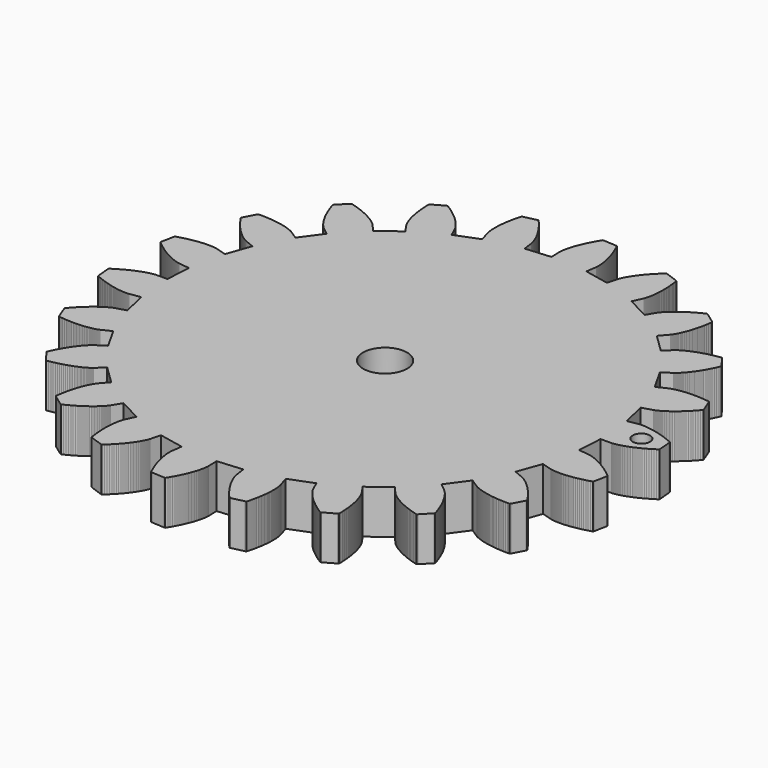
from build123d import *

# Parameters (mm, degrees)
F0_R     = 2.5
F1_DEPTH = 5


# Not quite as in the source:
# - the dataset's text gives a spline's control points without its knots; the knots are read off the source's solid


with BuildPart() as f1:
    # F0 (on Top) → F1 (new body)
    with BuildSketch(Plane.XY):
        Polygon((26.3997478077, -0.4197545319), (26.5654568077, 2.4303734681), (27.7857098077, 2.4303734681), (27.7960448077, 2.4307174681), (27.8132698077, 2.4314064681), (27.8363528077, 2.4327844681), (27.8663248077, 2.4348524681), (27.9024978077, 2.4382974681), (27.9452178077, 2.4427754681), (27.9944818077, 2.4486324681), (28.0499478077, 2.4562114681), (28.1116158077, 2.4658574681), (28.1794838077, 2.4772264681), (28.2535538077, 2.4910074681), (28.3341688077, 2.5071994681), (28.4202958077, 2.5264914681), (28.5129688077, 2.5481954681), (28.6111548077, 2.5730004681), (28.7155408077, 2.6012504681), (28.8254388077, 2.6326004681), (28.9411948077, 2.6677404681), (29.0628068077, 2.7070144681), (29.1895858077, 2.7500784681), (29.3218778077, 2.7972764681), (29.4596818077, 2.8489524681), (29.6026528077, 2.9051074681), (29.7507918077, 2.9657414681), (29.9037538077, 3.0315424681), (30.0615398077, 3.1025114681), (30.2241478077, 3.1786484681), (30.3912348077, 3.2602964681), (30.5631458077, 3.3474574681), (30.7388448077, 3.4404754681), (30.9193678077, 3.5393494681), (31.1036808077, 3.6440804681), (31.2917828077, 3.7550124681), (31.4840198077, 3.8724904681), (31.6793568077, 3.9965134681), (31.8784828077, 4.1270824681), (31.8850288077, 4.2528284681), (31.7627278077, 5.6880554681), (31.7355118077, 5.8107014681), (31.5170928077, 5.9061304681), (31.3034968077, 5.9950134681), (31.0943788077, 6.0783854681), (30.8900848077, 6.1562444681), (30.6906138077, 6.2285914681), (30.4963108077, 6.2954264681), (30.3071748077, 6.3574374681), (30.1232068077, 6.4142814681), (29.9444058077, 6.4663024681), (29.7714628077, 6.5141894681), (29.6040308077, 6.5572534681), (29.4421118077, 6.5965274681), (29.2857038077, 6.6313224681), (29.1354978077, 6.6626734681), (28.9911488077, 6.6902334681), (28.8526558077, 6.7143494681), (28.7203638077, 6.7353644681), (28.5939288077, 6.7536234681), (28.4740398077, 6.7687824681), (28.3603518077, 6.7811844681), (28.2528648077, 6.7911754681), (28.1515788077, 6.7990994681), (28.0568388077, 6.8049554681), (27.9682998077, 6.8090894681), (27.8863058077, 6.8115014681), (27.8108588077, 6.8128794681), (27.7419568077, 6.8128794681), (27.6796008077, 6.8115014681), (27.6237898077, 6.8097784681), (27.5741808077, 6.8073674681), (27.5314618077, 6.8046114681), (27.4949438077, 6.8018554681), (27.4653158077, 6.7987544681), (27.4418888077, 6.7963424681), (27.4253528077, 6.7939314681), (27.4150168077, 6.7925534681), (26.2119898077, 6.5865364681), (25.5677568077, 9.3681064681), (26.7387448077, 9.7119274681), (26.7487358077, 9.7150274681), (26.7645828077, 9.7205394681), (26.7866318077, 9.7284634681), (26.8148818077, 9.7387984681), (26.8486438077, 9.7522344681), (26.8886068077, 9.7687714681), (26.9337378077, 9.7880634681), (26.9850688077, 9.8111454681), (27.0415688077, 9.8376734681), (27.1035808077, 9.8679904681), (27.1707598077, 9.9020964681), (27.2431068077, 9.9403374681), (27.3206218077, 9.9827114681), (27.4033038077, 10.0299094681), (27.4908088077, 10.0812414681), (27.5827938077, 10.1377414681), (27.6796008077, 10.1990634681), (27.7808858077, 10.2655544681), (27.8863058077, 10.3368674681), (27.9958598077, 10.4140374681), (28.1095488077, 10.4967194681), (28.2270258077, 10.5849144681), (28.3482938077, 10.6789654681), (28.4733508077, 10.7792174681), (28.6015078077, 10.8853264681), (28.7331108077, 10.9979814681), (28.8674698077, 11.1168374681), (29.0049288077, 11.2422384681), (29.1451438077, 11.3741854681), (29.2877708077, 11.5130234681), (29.4331538077, 11.6587504681), (29.5802598077, 11.8110234681), (29.7297768077, 11.9708764681), (29.8810168077, 12.1376184681), (30.0336338077, 12.3115964681), (30.1876298077, 12.4931524681), (30.1583468077, 12.6151094681), (29.6371038077, 13.9583514681), (29.5761258077, 14.0682504681), (29.3397918077, 14.0978784681), (29.1096598077, 14.1233724681), (28.8857288077, 14.1443874681), (28.6676538077, 14.1616124681), (28.4561248077, 14.1747034681), (28.2507978077, 14.1840054681), (28.0516708077, 14.1902064681), (27.8590898077, 14.1929624681), (27.6730548077, 14.1926184681), (27.4935658077, 14.1895174681), (27.3206218077, 14.1840054681), (27.1542238077, 14.1757374681), (26.9947158077, 14.1654024681), (26.8414088077, 14.1529994681), (26.6953368077, 14.1388744681), (26.5554658077, 14.1230274681), (26.4228298077, 14.1058024681), (26.2963948077, 14.0875434681), (26.1768498077, 14.0682504681), (26.0641948077, 14.0482684681), (25.9584308077, 14.0275984681), (25.8588678077, 14.0069274681), (25.7661948077, 13.9855684681), (25.6804118077, 13.9648974681), (25.6011748077, 13.9442274681), (25.5284828077, 13.9239004681), (25.4623368077, 13.9042634681), (25.4027368077, 13.8856604681), (25.3493378077, 13.8680904681), (25.3028288077, 13.8518984681), (25.2625218077, 13.8374294681), (25.2284148077, 13.8243374681), (25.2005098077, 13.8129684681), (25.1791498077, 13.8040114681), (25.1636468077, 13.7971214681), (25.1540008077, 13.7929874681), (24.0577718077, 13.2562414681), (22.6559618077, 15.7436004681), (23.6829448077, 16.4033364681), (23.6915578077, 16.4095374681), (23.7053388077, 16.4191834681), (23.7242868077, 16.4329644681), (23.7480578077, 16.4508784681), (23.7769968077, 16.4732714681), (23.8104138077, 16.5001434681), (23.8486548077, 16.5314934681), (23.8910288077, 16.5680114681), (23.9378818077, 16.6093524681), (23.9888698077, 16.6558614681), (24.0436468077, 16.7075384681), (24.1025578077, 16.7647264681), (24.1649138077, 16.8274274681), (24.2310598077, 16.8956404681), (24.3003068077, 16.9697094681), (24.3726538077, 17.0496364681), (24.4481008077, 17.1357634681), (24.5266488077, 17.2280924681), (24.6076088077, 17.3266214681), (24.6913248077, 17.4313524681), (24.7767628077, 17.5426294681), (24.8649578077, 17.6604514681), (24.9545298077, 17.7848194681), (25.0461698077, 17.9164224681), (25.1395318077, 18.0542254681), (25.2339268077, 18.1992644681), (25.3293568077, 18.3511934681), (25.4261638077, 18.5103564681), (25.5233148077, 18.6764104681), (25.6211558077, 18.8496984681), (25.7193408077, 19.0305664681), (25.8178708077, 19.2183234681), (25.9160558077, 19.4136604681), (26.0142418077, 19.6162324681), (26.1117378077, 19.8263834681), (26.2085448077, 20.0437684681), (26.1461888077, 20.1526334681), (25.2673448077, 21.2943384681), (25.1781168077, 21.3828774681), (24.9428168077, 21.3446364681), (24.7147518077, 21.3043294681), (24.4939208077, 21.2612654681), (24.2799798077, 21.2161344681), (24.0732748077, 21.1692814681), (23.8734588077, 21.1203604681), (23.6808778077, 21.0704074681), (23.4951878077, 21.0187304681), (23.3167318077, 20.9660204681), (23.1455108077, 20.9126214681), (22.9811788077, 20.8581894681), (22.8240828077, 20.8034124681), (22.6735318077, 20.7486354681), (22.5302158077, 20.6938584681), (22.3937908077, 20.6387364681), (22.2642548077, 20.5843044681), (22.1416098077, 20.5305604681), (22.0255098077, 20.4775064681), (21.9166448077, 20.4251404681), (21.8139808077, 20.3741534681), (21.7182068077, 20.3245434681), (21.6286348077, 20.2766574681), (21.5456078077, 20.2301484681), (21.4691268077, 20.1860514681), (21.3988468077, 20.1436764681), (21.3347678077, 20.1037134681), (21.2768908077, 20.0665064681), (21.2248698077, 20.0317104681), (21.1787058077, 20.0000154681), (21.1387418077, 19.9714214681), (21.1039468077, 19.9459274681), (21.0750078077, 19.9238794681), (21.0515808077, 19.9052754681), (21.0333218077, 19.8904614681), (21.0205758077, 19.8794374681), (21.0126518077, 19.8725474681), (20.1121038077, 19.0491694681), (18.0664058077, 21.0407794681), (18.8653238077, 21.9630314681), (18.8718698077, 21.9712994681), (18.8825488077, 21.9843904681), (18.8970188077, 22.0029944681), (18.9145888077, 22.0271104681), (18.9359478077, 22.0563934681), (18.9607528077, 22.0918774681), (18.9883138077, 22.1325294681), (19.0186308077, 22.1793834681), (19.0520478077, 22.2324374681), (19.0878768077, 22.2913484681), (19.1261178077, 22.3564614681), (19.1664248077, 22.4277744681), (19.2084548077, 22.5056334681), (19.2525528077, 22.5896944681), (19.2983718077, 22.6803004681), (19.3452258077, 22.7774514681), (19.3934568077, 22.8814934681), (19.4427218077, 22.9920814681), (19.4926758077, 23.1092144681), (19.5433188077, 23.2335824681), (19.5943058077, 23.3644964681), (19.6452938077, 23.5022994681), (19.6966248077, 23.6469934681), (19.7476128077, 23.7985784681), (19.7979108077, 23.9573974681), (19.8475208077, 24.1231064681), (19.8964408077, 24.2957054681), (19.9446718077, 24.4755394681), (19.9911808077, 24.6626084681), (20.0363118077, 24.8562224681), (20.0793758077, 25.0574164681), (20.1210608077, 25.2654994681), (20.1603348077, 25.4804734681), (20.1971978077, 25.7023374681), (20.2316488077, 25.9314364681), (20.2633438077, 26.1674254681), (20.1727378077, 26.2542424681), (19.0076058077, 27.1020804681), (18.8973628077, 27.1616804681), (18.6823888077, 27.0590164681), (18.4749948077, 26.9560084681), (18.2751788077, 26.8526554681), (18.0825978077, 26.7489574681), (17.8972518077, 26.6456054681), (17.7194848077, 26.5425964681), (17.5489528077, 26.4402774681), (17.3853108077, 26.3383024681), (17.2289038077, 26.2377054681), (17.0797308077, 26.1381424681), (16.9371038077, 26.0396124681), (16.8017118077, 25.9428054681), (16.6728648077, 25.8477204681), (16.5509088077, 25.7547034681), (16.4354978077, 25.6637524681), (16.3262888077, 25.5748694681), (16.2239688077, 25.4887424681), (16.1275068077, 25.4050264681), (16.0375898077, 25.3240664681), (15.9535288077, 25.2465514681), (15.8753258077, 25.1717934681), (15.8033228077, 25.1004794681), (15.7368328077, 25.0326114681), (15.6758538077, 24.9685324681), (15.6203878077, 24.9082434681), (15.5700898077, 24.8520884681), (15.5249588077, 24.7997224681), (15.4846518077, 24.7518364681), (15.4495118077, 24.7084274681), (15.4191948077, 24.6694984681), (15.3930118077, 24.6353914681), (15.3716528077, 24.6061084681), (15.3540828077, 24.5816484681), (15.3409908077, 24.5623554681), (15.3316888077, 24.5482304681), (15.3258328077, 24.5396184681), (14.6936578077, 23.4954094681), (12.1697808077, 24.8300394681), (12.6768988077, 25.9403944681), (12.6810328077, 25.9496954681), (12.6872338077, 25.9655434681), (12.6958468077, 25.9872474681), (12.7061818077, 26.0154974681), (12.7182398077, 26.0496034681), (12.7320198077, 26.0902554681), (12.7468338077, 26.1374534681), (12.7630258077, 26.1911964681), (12.7799068077, 26.2511414681), (12.7978218077, 26.3179764681), (12.8160808077, 26.3910124681), (12.8346838077, 26.4709384681), (12.8532878077, 26.5574104681), (12.8718908077, 26.6504284681), (12.8901498077, 26.7503354681), (12.9077198077, 26.8567894681), (12.9249458077, 26.9701334681), (12.9407928077, 27.0900224681), (12.9559518077, 27.2168014681), (12.9693868077, 27.3501274681), (12.9814448077, 27.4899974681), (12.9917808077, 27.6367594681), (13.0000488077, 27.7900654681), (13.0059048077, 27.9499184681), (13.0096948077, 28.1166604681), (13.0107288077, 28.2896044681), (13.0090058077, 28.4690944681), (13.0041828077, 28.6551294681), (12.9962588077, 28.8473654681), (12.9848898077, 29.0461474681), (12.9700758077, 29.2511304681), (12.9511278077, 29.4623154681), (12.9283908077, 29.6800454681), (12.9011748077, 29.9032874681), (12.8698238077, 30.1327304681), (12.8336508077, 30.3680304681), (12.7220298077, 30.4259084681), (11.3656958077, 30.9113224681), (11.2427058077, 30.9371604681), (11.0652828077, 30.7783414681), (10.8954398077, 30.6209004681), (10.7328308077, 30.4655264681), (10.5771128077, 30.3118754681), (10.4286298077, 30.1606364681), (10.2870358077, 30.0114634681), (10.1523328077, 29.8650464681), (10.0238308077, 29.7213864681), (9.9022188077, 29.5804814681), (9.7871528077, 29.4430224681), (9.6782878077, 29.3083194681), (9.5752788077, 29.1774054681), (9.4784718077, 29.0499374681), (9.3878658077, 28.9262584681), (9.3027718077, 28.8063684681), (9.2231908077, 28.6906134681), (9.1491208077, 28.5786484681), (9.0802188077, 28.4715054681), (9.0164848077, 28.3684974681), (8.9579178077, 28.2703124681), (8.9038298077, 28.1766054681), (8.8549098077, 28.0877224681), (8.8101238077, 28.0040064681), (8.7694718077, 27.9254584681), (8.7332978077, 27.8517334681), (8.7009138077, 27.7838644681), (8.6723198077, 27.7208194681), (8.6475148077, 27.6636304681), (8.6258108077, 27.6119544681), (8.6075518077, 27.5661344681), (8.5923938077, 27.5261714681), (8.5799908077, 27.4917204681), (8.5700008077, 27.4634704681), (8.5627658077, 27.4414224681), (8.5579428077, 27.4248854681), (8.5548418077, 27.4152394681), (8.2423718077, 26.2352944681), (5.4449538077, 26.8047684681), (5.6185868077, 28.0126184681), (5.6196208077, 28.0229544681), (5.6213428077, 28.0398354681), (5.6234098077, 28.0632614681), (5.6254768077, 28.0932344681), (5.6275438077, 28.1294074681), (5.6289228077, 28.1724714681), (5.6299558077, 28.2217364681), (5.6303008077, 28.2778914681), (5.6299558077, 28.3402474681), (5.6282338077, 28.4091494681), (5.6247878077, 28.4845974681), (5.6203098077, 28.5665904681), (5.6137638077, 28.6547844681), (5.6054958077, 28.7491804681), (5.5948158077, 28.8501214681), (5.5817248077, 28.9572644681), (5.5662218077, 29.0709524681), (5.5476178077, 29.1904974681), (5.5262588077, 29.3162434681), (5.5017978077, 29.4478454681), (5.4738928077, 29.5856494681), (5.4425428077, 29.7293104681), (5.4074028077, 29.8784824681), (5.3681288077, 30.0338564681), (5.3247208077, 30.1947424681), (5.2768338077, 30.3607964681), (5.2248128077, 30.5327064681), (5.1679688077, 30.7097844681), (5.1059568077, 30.8923744681), (5.0391218077, 31.0797874681), (4.9667748077, 31.2723684681), (4.8892608077, 31.4694274681), (4.8062338077, 31.6716544681), (4.7173498077, 31.8783604681), (4.6222658077, 32.0898894681), (4.5213238077, 32.3055524681), (4.3979898077, 32.3293234681), (2.9596628077, 32.4130394681), (2.8346058077, 32.4033934681), (2.7092038077, 32.2008214681), (2.5903478077, 32.0020394681), (2.4783828077, 31.8070474681), (2.3722738077, 31.6158444681), (2.2723658077, 31.4287754681), (2.1783148077, 31.2458414681), (2.0901198077, 31.0673854681), (2.0077828077, 30.8934074681), (1.9306128077, 30.7239094681), (1.8589548077, 30.5592334681), (1.7921198077, 30.3997254681), (1.7304518077, 30.2450404681), (1.6736078077, 30.0955234681), (1.6212428077, 29.9511744681), (1.5733558077, 29.8119924681), (1.5299478077, 29.6786674681), (1.4899848077, 29.5505094681), (1.4544998077, 29.4282084681), (1.4224608077, 29.3114194681), (1.3935218077, 29.2004874681), (1.3683728077, 29.0957564681), (1.3459798077, 28.9965384681), (1.3266868077, 28.9035204681), (1.3101508077, 28.8167044681), (1.2960258077, 28.7360894681), (1.2843128077, 28.6613304681), (1.2743218077, 28.5931174681), (1.2667428077, 28.5311054681), (1.2605408077, 28.4756394681), (1.2557178077, 28.4263744681), (1.2526178077, 28.3836554681), (1.2502058077, 28.3471374681), (1.2488278077, 28.3171654681), (1.2481388077, 28.2937384681), (1.2477948077, 28.2768574681), (1.2481388077, 28.2665224681), (1.2805228077, 27.0466144681), (-1.5640921923, 26.8047684681), (-1.7380701923, 28.0126184681), (-1.7397921923, 28.0229544681), (-1.7428931923, 28.0394904681), (-1.7473711923, 28.0625724681), (-1.7539171923, 28.0918564681), (-1.7621851923, 28.1273404681), (-1.7728651923, 28.1690264681), (-1.7856121923, 28.2165684681), (-1.8011151923, 28.2703124681), (-1.8193741923, 28.3302564681), (-1.8403891923, 28.3957134681), (-1.8645051923, 28.4673714681), (-1.8920651923, 28.5445414681), (-1.9234161923, 28.6272244681), (-1.9578671923, 28.7157624681), (-1.9964521923, 28.8094694681), (-2.0391711923, 28.9086884681), (-2.0860241923, 29.0130744681), (-2.1373561923, 29.1226284681), (-2.1935111923, 29.2373504681), (-2.2541451923, 29.3568954681), (-2.3196021923, 29.4812634681), (-2.3902261923, 29.6101094681), (-2.4663631923, 29.7434344681), (-2.5476671923, 29.8812384681), (-2.6344841923, 30.0235214681), (-2.7271571923, 30.1695934681), (-2.8256861923, 30.3197994681), (-2.9300731923, 30.4737954681), (-3.0410051923, 30.6312364681), (-3.1577941923, 30.7921224681), (-3.2814721923, 30.9567974681), (-3.4113531923, 31.1242294681), (-3.5481231923, 31.2947614681), (-3.6917831923, 31.4680494681), (-3.8423341923, 31.6440944681), (-4.0001191923, 31.8225504681), (-4.1251761923, 31.8108364681), (-5.5287081923, 31.4856194681), (-5.6461861923, 31.4411774681), (-5.7092311923, 31.2117344681), (-5.7671091923, 30.9874584681), (-5.8198191923, 30.7686954681), (-5.8677061923, 30.5550994681), (-5.9107691923, 30.3477044681), (-5.9493541923, 30.1458224681), (-5.9838051923, 29.9494514681), (-6.0141221923, 29.7592824681), (-6.0403051923, 29.5753144681), (-6.0626981923, 29.3968584681), (-6.0816461923, 29.2249484681), (-6.0971491923, 29.0592384681), (-6.1098961923, 28.8997314681), (-6.1191981923, 28.7464244681), (-6.1260881923, 28.5996634681), (-6.1302221923, 28.4591034681), (-6.1322891923, 28.3250894681), (-6.1319441923, 28.1976204681), (-6.1298771923, 28.0766974681), (-6.1260881923, 27.9623204681), (-6.1209201923, 27.8544894681), (-6.1143741923, 27.7532034681), (-6.1067951923, 27.6584634681), (-6.0981831923, 27.5702684681), (-6.0888811923, 27.4889644681), (-6.0792341923, 27.4138614681), (-6.0692441923, 27.3456484681), (-6.0595971923, 27.2843254681), (-6.0496071923, 27.2292044681), (-6.0403051923, 27.1806284681), (-6.0313481923, 27.1385984681), (-6.0234241923, 27.1031134681), (-6.0161891923, 27.0738304681), (-6.0103331923, 27.0510924681), (-6.0058541923, 27.0349004681), (-6.0030981923, 27.0249104681), (-5.6279271923, 25.8635684681), (-8.2892631923, 24.8300394681), (-8.7963811923, 25.9400494681), (-8.8008601923, 25.9496954681), (-8.8087841923, 25.9648544681), (-8.8194631923, 25.9855244681), (-8.8339331923, 26.0117074681), (-8.8518471923, 26.0434024681), (-8.8738961923, 26.0802644681), (-8.8997341923, 26.1222954681), (-8.9297061923, 26.1694924681), (-8.9638131923, 26.2218584681), (-9.0023981923, 26.2790464681), (-9.0458061923, 26.3407144681), (-9.0940381923, 26.4068594681), (-9.1474371923, 26.4778284681), (-9.2056591923, 26.5525874681), (-9.2690481923, 26.6318244681), (-9.3379501923, 26.7151964681), (-9.4123641923, 26.8020124681), (-9.4922911923, 26.8926184681), (-9.5784181923, 26.9870144681), (-9.6704021923, 27.0845104681), (-9.7682431923, 27.1851074681), (-9.8722851923, 27.2891484681), (-9.9828721923, 27.3956024681), (-10.0996611923, 27.5051564681), (-10.2229951923, 27.6167774681), (-10.3532201923, 27.7311544681), (-10.4899901923, 27.8472544681), (-10.6336511923, 27.9654214681), (-10.7842011923, 28.0856544681), (-10.9419871923, 28.2069224681), (-11.1066621923, 28.3299124681), (-11.2785731923, 28.4542804681), (-11.4580621923, 28.5789924681), (-11.6444421923, 28.7050834681), (-11.8384011923, 28.8315184681), (-12.0399391923, 28.9582974681), (-12.1567271923, 28.9117884681), (-13.4121201923, 28.2045104681), (-13.5120281923, 28.1287184681), (-13.5078941923, 27.8906624681), (-13.5003151923, 27.6591524681), (-13.4892901923, 27.4345314681), (-13.4751651923, 27.2161124681), (-13.4579401923, 27.0049284681), (-13.4383031923, 26.8002894681), (-13.4159101923, 26.6025414681), (-13.3911051923, 26.4113384681), (-13.3645781923, 26.2273704681), (-13.3359841923, 26.0499484681), (-13.3056671923, 25.8797604681), (-13.2739721923, 25.7161184681), (-13.2408991923, 25.5597104681), (-13.2067931923, 25.4098494681), (-13.1719971923, 25.2668774681), (-13.1365131923, 25.1311414681), (-13.1006841923, 25.0019504681), (-13.0645101923, 24.8796494681), (-13.0283371923, 24.7642384681), (-12.9925081923, 24.6553734681), (-12.9570231923, 24.5533984681), (-12.9222281923, 24.4579694681), (-12.8884661923, 24.3694304681), (-12.8553931923, 24.2870924681), (-12.8236981923, 24.2116454681), (-12.7933811923, 24.1427434681), (-12.7644421923, 24.0800424681), (-12.7375711923, 24.0235424681), (-12.7127661923, 23.9735894681), (-12.6900281923, 23.9294914681), (-12.6697021923, 23.8915954681), (-12.6517881923, 23.8599004681), (-12.6369741923, 23.8340624681), (-12.6249161923, 23.8140814681), (-12.6159591923, 23.7996114681), (-12.6101021923, 23.7909984681), (-11.9231501923, 22.7822744681), (-14.1855441923, 21.0407794681), (-14.9848061923, 21.9630314681), (-14.9920411923, 21.9706104681), (-15.0037541923, 21.9830124681), (-15.0199461923, 21.9998934681), (-15.0409611923, 22.0209084681), (-15.0671441923, 22.0464024681), (-15.0988391923, 22.0756854681), (-15.1353571923, 22.1087584681), (-15.1773871923, 22.1456214681), (-15.2249291923, 22.1862734681), (-15.2783281923, 22.2300264681), (-15.3372401923, 22.2768794681), (-15.4020071923, 22.3268334681), (-15.4729761923, 22.3798874681), (-15.5501461923, 22.4353534681), (-15.6335181923, 22.4935754681), (-15.7227461923, 22.5538654681), (-15.8188641923, 22.6165654681), (-15.9211831923, 22.6809894681), (-16.0303931923, 22.7471354681), (-16.1458031923, 22.8146584681), (-16.2681041923, 22.8839054681), (-16.3972951923, 22.9541854681), (-16.5333771923, 23.0254984681), (-16.6763481923, 23.0971564681), (-16.8262101923, 23.1698484681), (-16.9833061923, 23.2425394681), (-17.1472931923, 23.3155754681), (-17.3185141923, 23.3886114681), (-17.4966251923, 23.4613034681), (-17.6823161923, 23.5336504681), (-17.8748971923, 23.6049634681), (-18.0750571923, 23.6755884681), (-18.2821071923, 23.7451794681), (-18.4967371923, 23.8133924681), (-18.7186011923, 23.8802264681), (-18.9477001923, 23.9449944681), (-19.0465741923, 23.8674804681), (-20.0515081923, 22.8353294681), (-20.1262671923, 22.7343884681), (-20.0552981923, 22.5070114681), (-19.9826061923, 22.2872144681), (-19.9088811923, 22.0746524681), (-19.8337781923, 21.8693244681), (-19.7576421923, 21.6712314681), (-19.6811601923, 21.4803734681), (-19.6039901923, 21.2967494681), (-19.5264761923, 21.1207054681), (-19.4489611923, 20.9515514681), (-19.3714461923, 20.7896314681), (-19.2946211923, 20.6346024681), (-19.2177951923, 20.4864634681), (-19.1423481923, 20.3455584681), (-19.0675891923, 20.2115444681), (-18.9938641923, 20.0844204681), (-18.9215171923, 19.9638424681), (-18.8505481923, 19.8501544681), (-18.7816461923, 19.7430114681), (-18.7144671923, 19.6424144681), (-18.6493541923, 19.5480194681), (-18.5866541923, 19.4601694681), (-18.5260201923, 19.3785204681), (-18.4684871923, 19.3030734681), (-18.4137101923, 19.2334824681), (-18.3620331923, 19.1700924681), (-18.3134581923, 19.1122144681), (-18.2683271923, 19.0601934681), (-18.2266411923, 19.0136854681), (-18.1884011923, 18.9726884681), (-18.1542941923, 18.9368594681), (-18.1243221923, 18.9061984681), (-18.0981391923, 18.8807044681), (-18.0764351923, 18.8600334681), (-18.0592101923, 18.8441864681), (-18.0468071923, 18.8331624681), (-18.0388831923, 18.8262714681), (-17.0952721923, 18.0521584681), (-18.7754451923, 15.7436004681), (-19.8024281923, 16.4033364681), (-19.8113851923, 16.4088484681), (-19.8258541923, 16.4174614681), (-19.8461811923, 16.4288294681), (-19.8723631923, 16.4432994681), (-19.9047471923, 16.4601804681), (-19.9433321923, 16.4794724681), (-19.9877741923, 16.5008324681), (-20.0384171923, 16.5246034681), (-20.0956051923, 16.5497524681), (-20.1589951923, 16.5769694681), (-20.2289311923, 16.6052184681), (-20.3050671923, 16.6351914681), (-20.3880941923, 16.6658524681), (-20.4776671923, 16.6975474681), (-20.5737851923, 16.7299314681), (-20.6767931923, 16.7623154681), (-20.7866921923, 16.7953884681), (-20.9027911923, 16.8284604681), (-21.0261261923, 16.8611894681), (-21.1560061923, 16.8935734681), (-21.2931211923, 16.9256124681), (-21.4367811923, 16.9566184681), (-21.5873321923, 16.9865904681), (-21.7447731923, 17.0151854681), (-21.9091041923, 17.0427454681), (-22.0799801923, 17.0682394681), (-22.2580921923, 17.0920104681), (-22.4430941923, 17.1140594681), (-22.6346411923, 17.1333514681), (-22.8327341923, 17.1505774681), (-23.0377171923, 17.1647024681), (-23.2495901923, 17.1760714681), (-23.4680091923, 17.1846834681), (-23.6929741923, 17.1895064681), (-23.9248291923, 17.1908854681), (-24.1628851923, 17.1888174681), (-24.2359211923, 17.0864984681), (-24.9094371923, 15.8128464681), (-24.9525011923, 15.6950244681), (-24.8205541923, 15.4969314681), (-24.6889511923, 15.3064174681), (-24.5580381923, 15.1231384681), (-24.4281581923, 14.9474384681), (-24.2996551923, 14.7786294681), (-24.1721871923, 14.6173984681), (-24.0464411923, 14.4630584681), (-23.9224181923, 14.3156084681), (-23.8004611923, 14.1750484681), (-23.6805721923, 14.0413784681), (-23.5630941923, 13.9145994681), (-23.4480281923, 13.7943654681), (-23.3353731923, 13.6803324681), (-23.2258191923, 13.5728454681), (-23.1193661923, 13.4715594681), (-23.0160131923, 13.3761304681), (-22.9161051923, 13.2869024681), (-22.8196421923, 13.2035314681), (-22.7269691923, 13.1260164681), (-22.6377411923, 13.0540144681), (-22.5529921923, 12.9871794681), (-22.4720321923, 12.9258564681), (-22.3955511923, 12.8697014681), (-22.3232041923, 12.8183694681), (-22.2556801923, 12.7722054681), (-22.1929801923, 12.7301754681), (-22.1347571923, 12.6929684681), (-22.0817031923, 12.6602394681), (-22.0338161923, 12.6316454681), (-21.9907521923, 12.6068404681), (-21.9532011923, 12.5861704681), (-21.9211621923, 12.5689444681), (-21.8946341923, 12.5551644681), (-21.8736191923, 12.5448294681), (-21.8581161923, 12.5375944681), (-21.8488151923, 12.5331154681), (-20.7253691923, 12.0563144681), (-21.6872401923, 9.3681064681), (-22.8582281923, 9.7119274681), (-22.8682181923, 9.7143384681), (-22.8847551923, 9.7184724681), (-22.9074921923, 9.7239854681), (-22.9367761923, 9.7301864681), (-22.9726051923, 9.7374204681), (-23.0149791923, 9.7450004681), (-23.0635551923, 9.7532684681), (-23.1190211923, 9.7615364681), (-23.1806881923, 9.7698044681), (-23.2492461923, 9.7777284681), (-23.3243491923, 9.7853074681), (-23.4059981923, 9.7925424681), (-23.4941921923, 9.7983994681), (-23.5892771923, 9.8035664681), (-23.6905631923, 9.8073564681), (-23.7983941923, 9.8101124681), (-23.9131161923, 9.8108014681), (-24.0340391923, 9.8094234681), (-24.1615071923, 9.8063224681), (-24.2955211923, 9.8008104681), (-24.4357371923, 9.7928864681), (-24.5824981923, 9.7818624681), (-24.7351161923, 9.7684264681), (-24.8942791923, 9.7515454681), (-25.0596441923, 9.7315644681), (-25.2312091923, 9.7081374681), (-25.4086321923, 9.6805764681), (-25.5919111923, 9.6495714681), (-25.7813911923, 9.6144314681), (-25.9763831923, 9.5748124681), (-26.1772331923, 9.5307154681), (-26.3835941923, 9.4821394681), (-26.5958121923, 9.4283954681), (-26.8128531923, 9.3698294681), (-27.0354061923, 9.3060944681), (-27.2634711923, 9.2368484681), (-27.3048121923, 9.1183374681), (-27.5921331923, 7.7065374681), (-27.6004011923, 7.5811354681), (-27.4178111923, 7.4281734681), (-27.2379771923, 7.2824454681), (-27.0609001923, 7.1436084681), (-26.8865781923, 7.0113164681), (-26.7157011923, 6.8859154681), (-26.5479251923, 6.7670594681), (-26.3839381923, 6.6544044681), (-26.2233971923, 6.5479514681), (-26.0666451923, 6.4473544681), (-25.9140271923, 6.3529594681), (-25.7655441923, 6.2644204681), (-25.6211941923, 6.1810484681), (-25.4813231923, 6.1035344681), (-25.3459311923, 6.0311874681), (-25.2150171923, 5.9640074681), (-25.0889271923, 5.9019964681), (-24.9680041923, 5.8444634681), (-24.8519041923, 5.7917534681), (-24.7409721923, 5.7431774681), (-24.6352081923, 5.6990804681), (-24.5349561923, 5.6591164681), (-24.4402151923, 5.6229434681), (-24.3509871923, 5.5905594681), (-24.2672721923, 5.5619654681), (-24.1894121923, 5.5364714681), (-24.1170651923, 5.5140784681), (-24.0509201923, 5.4947854681), (-23.9906301923, 5.4782494681), (-23.9365421923, 5.4641244681), (-23.8886561923, 5.4527554681), (-23.8466251923, 5.4431094681), (-23.8107961923, 5.4355304681), (-23.7815131923, 5.4300184681), (-23.7584311923, 5.4258834681), (-23.7418951923, 5.4234724681), (-23.7315591923, 5.4217494681), (-22.5192301923, 5.2805004681), (-22.6845951923, 2.4303734681), (-23.9051921923, 2.4303734681), (-23.9155271923, 2.4300284681), (-23.9324081923, 2.4293394681), (-23.9558351923, 2.4279614681), (-23.9858071923, 2.4258944681), (-24.0219811923, 2.4224494681), (-24.0647001923, 2.4179714681), (-24.1139651923, 2.4121144681), (-24.1690861923, 2.4045354681), (-24.2310981923, 2.3948884681), (-24.2989661923, 2.3835204681), (-24.3730361923, 2.3697394681), (-24.4536511923, 2.3532034681), (-24.5397791923, 2.3342554681), (-24.6324521923, 2.3125514681), (-24.7306371923, 2.2877464681), (-24.8350231923, 2.2594964681), (-24.9449221923, 2.2281464681), (-25.0606771923, 2.1930064681), (-25.1822891923, 2.1537324681), (-25.3090681923, 2.1106684681), (-25.4413601923, 2.0634704681), (-25.5791641923, 2.0117944681), (-25.7221351923, 1.9556394681), (-25.8699301923, 1.8946614681), (-26.0228921923, 1.8292044681), (-26.1810221923, 1.7582354681), (-26.3436311923, 1.6820984681), (-26.5107181923, 1.6004494681), (-26.6826281923, 1.5132894681), (-26.8583281923, 1.4202714681), (-27.0388511923, 1.3213974681), (-27.2231641923, 1.2166664681), (-27.4112661923, 1.1057344681), (-27.6031581923, 0.9879114681), (-27.7988391923, 0.8642334681), (-27.9979651923, 0.7336634681), (-28.0041671923, 0.6079174681), (-27.8822101923, -0.8276535319), (-27.8549941923, -0.9502985319), (-27.6365751923, -1.0453835319), (-27.4229791923, -1.1346115319), (-27.2138621923, -1.2176385319), (-27.0095681923, -1.2954975319), (-26.8100971923, -1.3678445319), (-26.6157931923, -1.4346795319), (-26.4266571923, -1.4966905319), (-26.2426891923, -1.5535345319), (-26.0638891923, -1.6059005319), (-25.8909451923, -1.6534425319), (-25.7235131923, -1.6965065319), (-25.5615941923, -1.7357805319), (-25.4051871923, -1.7705765319), (-25.2549801923, -1.8019265319), (-25.1106311923, -1.8294875319), (-24.9721381923, -1.8539475319), (-24.8398461923, -1.8749625319), (-24.7134111923, -1.8928765319), (-24.5935221923, -1.9080355319), (-24.4798341923, -1.9204375319), (-24.3723471923, -1.9307725319), (-24.2710611923, -1.9383525319), (-24.1763211923, -1.9445535319), (-24.0877821923, -1.9483425319), (-24.0057891923, -1.9510995319), (-23.9303411923, -1.9521325319), (-23.8614391923, -1.9521325319), (-23.7990831923, -1.9507545319), (-23.7432731923, -1.9490315319), (-23.6936631923, -1.9466205319), (-23.6509441923, -1.9438645319), (-23.6144261923, -1.9411085319), (-23.5847981923, -1.9380075319), (-23.5613721923, -1.9355965319), (-23.5448351923, -1.9331845319), (-23.5345001923, -1.9318065319), (-22.3314721923, -1.7257895319), (-21.6872401923, -4.5073595319), (-22.8582281923, -4.8511805319), (-22.8682181923, -4.8542805319), (-22.8840661923, -4.8597935319), (-22.9061141923, -4.8677165319), (-22.9343641923, -4.8783965319), (-22.9681261923, -4.8914885319), (-23.0077451923, -4.9080245319), (-23.0532201923, -4.9273175319), (-23.1042071923, -4.9503995319), (-23.1610511923, -4.9769265319), (-23.2230631923, -5.0072435319), (-23.2902431923, -5.0413495319), (-23.3625901923, -5.0795905319), (-23.4401041923, -5.1219645319), (-23.5227861923, -5.1691625319), (-23.6102921923, -5.2204945319), (-23.7022761923, -5.2769945319), (-23.7990831923, -5.3383165319), (-23.9003691923, -5.4048075319), (-24.0057891923, -5.4764655319), (-24.1153431923, -5.5532905319), (-24.2290311923, -5.6359735319), (-24.3465091923, -5.7241675319), (-24.4677761923, -5.8182185319), (-24.5928331923, -5.9184705319), (-24.7209911923, -6.0249245319), (-24.8525931923, -6.1372345319), (-24.9869521923, -6.2560905319), (-25.1244111923, -6.3814915319), (-25.2646271923, -6.5134385319), (-25.4072541923, -6.6522765319), (-25.5526371923, -6.7980035319), (-25.6997421923, -6.9502775319), (-25.8492591923, -7.1101295319), (-26.0001551923, -7.2768725319), (-26.1531171923, -7.4508495319), (-26.3071131923, -7.6324055319), (-26.2778291923, -7.7547065319), (-25.7565861923, -9.0976055319), (-25.6956081923, -9.2075035319), (-25.4592751923, -9.2371315319), (-25.2291421923, -9.2626255319), (-25.0052111923, -9.2836405319), (-24.7871361923, -9.3008655319), (-24.5756081923, -9.3139575319), (-24.3702801923, -9.3232585319), (-24.1711531923, -9.3294605319), (-23.9785731923, -9.3322165319), (-23.7925371923, -9.3318715319), (-23.6130481923, -9.3287705319), (-23.4401041923, -9.3232585319), (-23.2737061923, -9.3149905319), (-23.1141981923, -9.3046555319), (-22.9608911923, -9.2922525319), (-22.8144751923, -9.2781285319), (-22.6749481923, -9.2622805319), (-22.5419681923, -9.2453995319), (-22.4158771923, -9.2267965319), (-22.2963321923, -9.2075035319), (-22.1836781923, -9.1875225319), (-22.0775691923, -9.1668515319), (-21.9783501923, -9.1461805319), (-21.8856771923, -9.1251655319), (-21.7998941923, -9.1041505319), (-21.7203121923, -9.0834805319), (-21.6479651923, -9.0631545319), (-21.5818201923, -9.0435175319), (-21.5218751923, -9.0249135319), (-21.4688211923, -9.0076885319), (-21.4223121923, -8.9911515319), (-21.3820041923, -8.9766825319), (-21.3478981923, -8.9635905319), (-21.3199921923, -8.9522225319), (-21.2986331923, -8.9432645319), (-21.2831301923, -8.9363745319), (-21.2734841923, -8.9322405319), (-20.1772541923, -8.3958395319), (-18.7754451923, -10.8828535319), (-19.8024281923, -11.5429335319), (-19.8110411923, -11.5487905319), (-19.8248211923, -11.5584365319), (-19.8437691923, -11.5722175319), (-19.8675401923, -11.5901315319), (-19.8964791923, -11.6125245319), (-19.9298961923, -11.6393965319), (-19.9681371923, -11.6707465319), (-20.0105121923, -11.7072645319), (-20.0573651923, -11.7486065319), (-20.1080081923, -11.7951145319), (-20.1631291923, -11.8467915319), (-20.2220401923, -11.9039795319), (-20.2843971923, -11.9666805319), (-20.3505431923, -12.0348935319), (-20.4197891923, -12.1089635319), (-20.4921361923, -12.1892335319), (-20.5675841923, -12.2750165319), (-20.6461321923, -12.3673455319), (-20.7270911923, -12.4658745319), (-20.8104631923, -12.5706055319), (-20.8962461923, -12.6818825319), (-20.9844401923, -12.7997045319), (-21.0740131923, -12.9244175319), (-21.1656521923, -13.0556755319), (-21.2586701923, -13.1934795319), (-21.3534101923, -13.3385175319), (-21.4488391923, -13.4904465319), (-21.5456461923, -13.6496095319), (-21.6427981923, -13.8156635319), (-21.7406391923, -13.9892965319), (-21.8388241923, -14.1698195319), (-21.9373541923, -14.3575765319), (-22.0355391923, -14.5529135319), (-22.1337241923, -14.7554855319), (-22.2312201923, -14.9656365319), (-22.3280271923, -15.1830215319), (-22.2653271923, -15.2918865319), (-21.3868271923, -16.4335915319), (-21.2972551923, -16.5221305319), (-21.0622991923, -16.4838895319), (-20.8342341923, -16.4435825319), (-20.6134031923, -16.4005185319), (-20.3994631923, -16.3553875319), (-20.1927571923, -16.3085345319), (-19.9929421923, -16.2596145319), (-19.8003611923, -16.2096605319), (-19.6146701923, -16.1579835319), (-19.4362141923, -16.1052735319), (-19.2649931923, -16.0518745319), (-19.1006621923, -15.9974425319), (-18.9432211923, -15.9430095319), (-18.7930151923, -15.8878885319), (-18.6496991923, -15.8331115319), (-18.5132731923, -15.7779895319), (-18.3837381923, -15.7235575319), (-18.2610921923, -15.6698135319), (-18.1449921923, -15.6167595319), (-18.0357831923, -15.5643935319), (-17.9334641923, -15.5134065319), (-17.8373451923, -15.4637975319), (-17.7481171923, -15.4159105319), (-17.6650911923, -15.3694015319), (-17.5886091923, -15.3253045319), (-17.5183301923, -15.2829295319), (-17.4542511923, -15.2433105319), (-17.3963731923, -15.2057595319), (-17.3443521923, -15.1709635319), (-17.2981881923, -15.1392695319), (-17.2578801923, -15.1106745319), (-17.2234291923, -15.0851815319), (-17.1944911923, -15.0631325319), (-17.1710641923, -15.0445285319), (-17.1528051923, -15.0297155319), (-17.1400581923, -15.0186905319), (-17.1321341923, -15.0118005319), (-16.2312421923, -14.1884225319), (-14.1855441923, -16.1800325319), (-14.9848061923, -17.1022845319), (-14.9913521923, -17.1105525319), (-15.0020321923, -17.1236445319), (-15.0161571923, -17.1422475319), (-15.0340711923, -17.1663635319), (-15.0554311923, -17.1956465319), (-15.0802351923, -17.2311315319), (-15.1077961923, -17.2717835319), (-15.1381131923, -17.3186365319), (-15.1715301923, -17.3716905319), (-15.2073591923, -17.4306025319), (-15.2456001923, -17.4957145319), (-15.2859081923, -17.5670275319), (-15.3279381923, -17.6448865319), (-15.3720351923, -17.7289475319), (-15.4178551923, -17.8195535319), (-15.4647081923, -17.9167055319), (-15.5129391923, -18.0207465319), (-15.5622041923, -18.1313345319), (-15.6121581923, -18.2484675319), (-15.6628011923, -18.3728355319), (-15.7137891923, -18.5037495319), (-15.7647761923, -18.6415535319), (-15.8161081923, -18.7862475319), (-15.8670951923, -18.9378315319), (-15.9173941923, -19.0966505319), (-15.9670031923, -19.2623595319), (-16.0159231923, -19.4353035319), (-16.0638101923, -19.6151375319), (-16.1106641923, -19.8018615319), (-16.1554501923, -19.9958205319), (-16.1988581923, -20.1966695319), (-16.2405441923, -20.4047525319), (-16.2798181923, -20.6197265319), (-16.3166801923, -20.8415915319), (-16.3511311923, -21.0706895319), (-16.3828261923, -21.3066785319), (-16.2918761923, -21.3934955319), (-15.1270891923, -22.2413335319), (-15.0165011923, -22.3009335319), (-14.8018721923, -22.1982695319), (-14.5944771923, -22.0952615319), (-14.3946611923, -21.9919085319), (-14.2020811923, -21.8885555319), (-14.0167341923, -21.7852025319), (-13.8389681923, -21.6821945319), (-13.6680911923, -21.5795305319), (-13.5047931923, -21.4779005319), (-13.3483861923, -21.3769585319), (-13.1988691923, -21.2773955319), (-13.0565861923, -21.1788655319), (-12.9208501923, -21.0820585319), (-12.7923481923, -20.9869745319), (-12.6703911923, -20.8939565319), (-12.5549801923, -20.8030065319), (-12.4457711923, -20.7141225319), (-12.3434521923, -20.6279955319), (-12.2469891923, -20.5442795319), (-12.1570721923, -20.4636645319), (-12.0730121923, -20.3858045319), (-11.9948081923, -20.3110465319), (-11.9228051923, -20.2397325319), (-11.8563151923, -20.1718645319), (-11.7953371923, -20.1077855319), (-11.7395261923, -20.0474965319), (-11.6895721923, -19.9913415319), (-11.6440971923, -19.9389765319), (-11.6041341923, -19.8910895319), (-11.5689941923, -19.8476815319), (-11.5386771923, -19.8087515319), (-11.5124951923, -19.7746455319), (-11.4911351923, -19.7453615319), (-11.4735651923, -19.7209015319), (-11.4604741923, -19.7016085319), (-11.4511721923, -19.6874845319), (-11.4453151923, -19.6788715319), (-10.8131401923, -18.6346625319), (-8.2892631923, -19.9692925319), (-8.7963811923, -21.0796475319), (-8.8005151923, -21.0889485319), (-8.8067171923, -21.1047965319), (-8.8153291923, -21.1265005319), (-8.8256651923, -21.1547505319), (-8.8377221923, -21.1888565319), (-8.8515031923, -21.2298535319), (-8.8663171923, -21.2767065319), (-8.8825091923, -21.3304505319), (-8.8993901923, -21.3903945319), (-8.9173041923, -21.4572295319), (-8.9355631923, -21.5302655319), (-8.9541671923, -21.6101915319), (-8.9727701923, -21.6966635319), (-8.9913741923, -21.7896815319), (-9.0096331923, -21.8895895319), (-9.0272031923, -21.9963875319), (-9.0440841923, -22.1093865319), (-9.0602761923, -22.2292755319), (-9.0750901923, -22.3560555319), (-9.0888701923, -22.4893805319), (-9.1009281923, -22.6292515319), (-9.1112631923, -22.7760125319), (-9.1191871923, -22.9293185319), (-9.1253881923, -23.0891715319), (-9.1291781923, -23.2559145319), (-9.1302111923, -23.4288575319), (-9.1284881923, -23.6083475319), (-9.1236651923, -23.7943825319), (-9.1157421923, -23.9866185319), (-9.1043731923, -24.1854005319), (-9.0892141923, -24.3903835319), (-9.0706111923, -24.6015685319), (-9.0478731923, -24.8192985319), (-9.0206571923, -25.0425405319), (-8.9893071923, -25.2719835319), (-8.9531331923, -25.5072835319), (-8.8415121923, -25.5651615319), (-7.4851781923, -26.0505755319), (-7.3621881923, -26.0767585319), (-7.1847661923, -25.9175945319), (-7.0149221923, -25.7601535319), (-6.8523141923, -25.6047805319), (-6.6965961923, -25.4511285319), (-6.5481121923, -25.2998895319), (-6.4065191923, -25.1507165319), (-6.2714711923, -25.0042995319), (-6.1433131923, -24.8606395319), (-6.0217011923, -24.7200795319), (-5.9066351923, -24.5822755319), (-5.7977701923, -24.4479175319), (-5.6947621923, -24.3166585319), (-5.5979551923, -24.1891905319), (-5.5070041923, -24.0655115319), (-5.4222551923, -23.9456225319), (-5.3426731923, -23.8298665319), (-5.2686041923, -23.7182455319), (-5.1997021923, -23.6107585319), (-5.1359671923, -23.5077505319), (-5.0774011923, -23.4095655319), (-5.0233131923, -23.3158585319), (-4.9743921923, -23.2269755319), (-4.9296061923, -23.1432595319), (-4.8889541923, -23.0647115319), (-4.8527801923, -22.9913305319), (-4.8203971923, -22.9231175319), (-4.7918021923, -22.8604175319), (-4.7669981923, -22.8028835319), (-4.7452941923, -22.7515525319), (-4.7270351923, -22.7053875319), (-4.7118761923, -22.6654245319), (-4.6994741923, -22.6309735319), (-4.6894831923, -22.6027235319), (-4.6822481923, -22.5806755319), (-4.6774251923, -22.5644835319), (-4.6743251923, -22.5544925319), (-4.3618541923, -21.3745475319), (-1.5640921923, -21.9440215319), (-1.7380701923, -23.1522165319), (-1.7391031923, -23.1625515319), (-1.7408261923, -23.1794325319), (-1.7428931923, -23.2025155319), (-1.7449601923, -23.2324875319), (-1.7466821923, -23.2690055319), (-1.7484051923, -23.3117245319), (-1.7494381923, -23.3613335319), (-1.7497831923, -23.4171445319), (-1.7494381923, -23.4795005319), (-1.7477161923, -23.5484025319), (-1.7442711923, -23.6238505319), (-1.7397921923, -23.7058435319), (-1.7332471923, -23.7940375319), (-1.7249781923, -23.8884335319), (-1.7142991923, -23.9893745319), (-1.7012071923, -24.0965175319), (-1.6857041923, -24.2102055319), (-1.6671011923, -24.3297505319), (-1.6457411923, -24.4554965319), (-1.6212811923, -24.5870985319), (-1.5933761923, -24.7249025319), (-1.5620251923, -24.8685635319), (-1.5265411923, -25.0180805319), (-1.4876111923, -25.1731095319), (-1.4442031923, -25.3339955319), (-1.3963161923, -25.5000495319), (-1.3442951923, -25.6719595319), (-1.2871071923, -25.8490375319), (-1.2254391923, -26.0316275319), (-1.1586051923, -26.2190405319), (-1.0862581923, -26.4116215319), (-1.0087431923, -26.6090255319), (-0.9257161923, -26.8109085319), (-0.8368331923, -27.0179585319), (-0.7417481923, -27.2291425319), (-0.6408071923, -27.4448055319), (-0.5174721923, -27.4689215319), (0.9208548077, -27.5522925319), (1.0462568077, -27.5426465319), (1.1713128077, -27.3400745319), (1.2901688077, -27.1412925319), (1.4021348077, -26.9463005319), (1.5082438077, -26.7550975319), (1.6081518077, -26.5680285319), (1.7022028077, -26.3850945319), (1.7903968077, -26.2066385319), (1.8727348077, -26.0326605319), (1.9499048077, -25.8631625319), (2.0215628077, -25.6988315319), (2.0883978077, -25.5389785319), (2.1500648077, -25.3842935319), (2.2069088077, -25.2347765319), (2.2592748077, -25.0904275319), (2.3071608077, -24.9512455319), (2.3509138077, -24.8179205319), (2.3905328077, -24.6897625319), (2.4263618077, -24.5674615319), (2.4584008077, -24.4506735319), (2.4869948077, -24.3397415319), (2.5121448077, -24.2350105319), (2.5345378077, -24.1357915319), (2.5538298077, -24.0427735319), (2.5703668077, -23.9559575319), (2.5844918077, -23.8753425319), (2.5962048077, -23.8005835319), (2.6061958077, -23.7323705319), (2.6137748077, -23.6703585319), (2.6199758077, -23.6148925319), (2.6247988077, -23.5656285319), (2.6278998077, -23.5229085319), (2.6303108077, -23.4863905319), (2.6316888077, -23.4564185319), (2.6323778077, -23.4329915319), (2.6327228077, -23.4161105319), (2.6327228077, -23.4057755319), (2.5999948077, -22.1858675319), (5.4449538077, -21.9440215319), (5.6185868077, -23.1518725319), (5.6203098077, -23.1622075319), (5.6234098077, -23.1787435319), (5.6278888077, -23.2018265319), (5.6344348077, -23.2311095319), (5.6427028077, -23.2665935319), (5.6533828077, -23.3082795319), (5.6661298077, -23.3558215319), (5.6816318077, -23.4095655319), (5.6998908077, -23.4695095319), (5.7209068077, -23.5349665319), (5.7450218077, -23.6066245319), (5.7729278077, -23.6837945319), (5.8039328077, -23.7664775319), (5.8383838077, -23.8550165319), (5.8769688077, -23.9490675319), (5.9196888077, -24.0479415319), (5.9665418077, -24.1523275319), (6.0182178077, -24.2622265319), (6.0740288077, -24.3766035319), (6.1346628077, -24.4961485319), (6.2001188077, -24.6205165319), (6.2710878077, -24.7493625319), (6.3468798077, -24.8826885319), (6.4281848077, -25.0204915319), (6.5150008077, -25.1627745319), (6.6076738077, -25.3088465319), (6.7062038077, -25.4590525319), (6.8105898077, -25.6130485319), (6.9215218077, -25.7704895319), (7.0386558077, -25.9313755319), (7.1619898077, -26.0960505319), (7.2918698077, -26.2634825319), (7.4286398077, -26.4340145319), (7.5723008077, -26.6073025319), (7.7228518077, -26.7833475319), (7.8806368077, -26.9618035319), (8.0056938077, -26.9500895319), (9.4092258077, -26.6252175319), (9.5267038077, -26.5804315319), (9.5897488077, -26.3509875319), (9.6476258077, -26.1267125319), (9.7003358077, -25.9079485319), (9.7482228077, -25.6943525319), (9.7912868077, -25.4869575319), (9.8298718077, -25.2850755319), (9.8643228077, -25.0887045319), (9.8946398077, -24.8985355319), (9.9208218077, -24.7145675319), (9.9432158077, -24.5364555319), (9.9621638077, -24.3642015319), (9.9776668077, -24.1984925319), (9.9904128077, -24.0389845319), (9.9997148077, -23.8856775319), (10.0066048077, -23.7389165319), (10.0107388077, -23.5983565319), (10.0128068077, -23.4643425319), (10.0124618077, -23.3368735319), (10.0103948077, -23.2159505319), (10.0069498077, -23.1015735319), (10.0014378077, -22.9937425319), (9.9948918077, -22.8924565319), (9.9873128077, -22.7977165319), (9.9786998077, -22.7095215319), (9.9697428077, -22.6282175319), (9.9600968077, -22.5534595319), (9.9501058077, -22.4852465319), (9.9401148077, -22.4235785319), (9.9301238077, -22.3684575319), (9.9208218077, -22.3198815319), (9.9118648077, -22.2778515319), (9.9039418077, -22.2423665319), (9.8967068077, -22.2130835319), (9.8908498077, -22.1906905319), (9.8863718077, -22.1741545319), (9.8836148077, -22.1641635319), (9.5084448077, -21.0028215319), (12.1697808077, -19.9692925319), (12.6768988077, -21.0793025319), (12.6813768077, -21.0889485319), (12.6893008077, -21.1041075319), (12.6999808077, -21.1247775319), (12.7144498077, -21.1509605319), (12.7327088077, -21.1826555319), (12.7544138077, -21.2195185319), (12.7802518077, -21.2615485319), (12.8102238077, -21.3087465319), (12.8443308077, -21.3611115319), (12.8832598077, -21.4183005319), (12.9263238077, -21.4799675319), (12.9745548077, -21.5461135319), (13.0279538077, -21.6170825319), (13.0861758077, -21.6918405319), (13.1495658077, -21.7710775319), (13.2184678077, -21.8544495319), (13.2928818077, -21.9412655319), (13.3731528077, -22.0322165319), (13.4589358077, -22.1262675319), (13.5509198077, -22.2237635319), (13.6487598077, -22.3247045319), (13.7528018077, -22.4284025319), (13.8633898077, -22.5352005319), (13.9801778077, -22.6444095319), (14.1035128077, -22.7560305319), (14.2337378077, -22.8704075319), (14.3705078077, -22.9865075319), (14.5141678077, -23.1046745319), (14.6647188077, -23.2249085319), (14.8225038077, -23.3461755319), (14.9871798077, -23.4691655319), (15.1590898077, -23.5935335319), (15.3385798077, -23.7185905319), (15.5249588077, -23.8443365319), (15.7189178077, -23.9707715319), (15.9208008077, -24.0975505319), (16.0372448077, -24.0510425319), (17.2926378077, -23.3437635319), (17.3925458077, -23.2679715319), (17.3884108077, -23.0299155319), (17.3808318077, -22.7984055319), (17.3698078077, -22.5737855319), (17.3556828077, -22.3553665319), (17.3384578077, -22.1441815319), (17.3188208077, -21.9395435319), (17.2964268077, -21.7417945319), (17.2719668077, -21.5505915319), (17.2450948077, -21.3666235319), (17.2165008077, -21.1892015319), (17.1861838077, -21.0190135319), (17.1544888077, -20.8553715319), (17.1214168077, -20.6989645319), (17.0873098077, -20.5491025319), (17.0525148077, -20.4061315319), (17.0170298077, -20.2703945319), (16.9812008077, -20.1412035319), (16.9450278077, -20.0189025319), (16.9091988077, -19.9034915319), (16.8730248077, -19.7946265319), (16.8378848077, -19.6926515319), (16.8027448077, -19.5972225319), (16.7689828077, -19.5086835319), (16.7359098077, -19.4266905319), (16.7042148077, -19.3508985319), (16.6738988077, -19.2819965319), (16.6449598077, -19.2192955319), (16.6180878077, -19.1627965319), (16.5932828077, -19.1128425319), (16.5705458077, -19.0687445319), (16.5502198077, -19.0311935319), (16.5323048077, -18.9991545319), (16.5174908077, -18.9733155319), (16.5054328077, -18.9533345319), (16.4964758077, -18.9388645319), (16.4909638077, -18.9302525319), (15.8036678077, -17.9215285319), (18.0664058077, -16.1800325319), (18.8656678077, -17.1022845319), (18.8725588077, -17.1098635319), (18.8842718077, -17.1222665319), (18.9004638077, -17.1391465319), (18.9218228077, -17.1601625319), (18.9480058077, -17.1856555319), (18.9793568077, -17.2149395319), (19.0158748077, -17.2480115319), (19.0579048077, -17.2848745319), (19.1054468077, -17.3255265319), (19.1588458077, -17.3692795319), (19.2177568077, -17.4161325319), (19.2825248077, -17.4660865319), (19.3534938077, -17.5191415319), (19.4306638077, -17.5746075319), (19.5140348077, -17.6328295319), (19.6036078077, -17.6931185319), (19.6993818077, -17.7558195319), (19.8017008077, -17.8202425319), (19.9109098077, -17.8863885319), (20.0263208077, -17.9539125319), (20.1486218077, -18.0231585319), (20.2778128077, -18.0934385319), (20.4138938077, -18.1647515319), (20.5568658077, -18.2364095319), (20.7067268077, -18.3091015319), (20.8638238077, -18.3817925319), (21.0278098077, -18.4548285319), (21.1990318077, -18.5278645319), (21.3771428077, -18.6005565319), (21.5628338077, -18.6729035319), (21.7554138077, -18.7442165319), (21.9555748077, -18.8151855319), (22.1626248077, -18.8844325319), (22.3772538077, -18.9526455319), (22.5991178077, -19.0194805319), (22.8282168077, -19.0842475319), (22.9270908077, -19.0067335319), (23.9320258077, -17.9745825319), (24.0067838077, -17.8736415319), (23.9358148077, -17.6462655319), (23.8631238077, -17.4264675319), (23.7893988077, -17.2139055319), (23.7142958077, -17.0085775319), (23.6381588077, -16.8104845319), (23.5616778077, -16.6196265319), (23.4845078077, -16.4363475319), (23.4069928077, -16.2599585319), (23.3294788077, -16.0908045319), (23.2519638077, -15.9288845319), (23.1751378077, -15.7738555319), (23.0986568077, -15.6257165319), (23.0228648077, -15.4848125319), (22.9481068077, -15.3507975319), (22.8743818077, -15.2236735319), (22.8020338077, -15.1030955319), (22.7310658077, -14.9894075319), (22.6621638077, -14.8822645319), (22.5949838077, -14.7816685319), (22.5298718077, -14.6872725319), (22.4671708077, -14.5994225319), (22.4068818077, -14.5177735319), (22.3490038077, -14.4423265319), (22.2942268077, -14.3727355319), (22.2425508077, -14.3093455319), (22.1939748077, -14.2514675319), (22.1488438077, -14.1994465319), (22.1071588077, -14.1529385319), (22.0689178077, -14.1119415319), (22.0348118077, -14.0761125319), (22.0048388077, -14.0457955319), (21.9786568077, -14.0199575319), (21.9569528077, -13.9996315319), (21.9397268077, -13.9837845319), (21.9273248077, -13.9724155319), (21.9194008077, -13.9655255319), (20.9757888077, -13.1914125319), (22.6559618077, -10.8828535319), (23.6829448077, -11.5425895319), (23.6919028077, -11.5481015319), (23.7063718077, -11.5567145319), (23.7266978077, -11.5680835319), (23.7532248077, -11.5825525319), (23.7852648077, -11.5994335319), (23.8238498077, -11.6187255319), (23.8682918077, -11.6400855319), (23.9189338077, -11.6638565319), (23.9761228077, -11.6890055319), (24.0395128077, -11.7162225319), (24.1094478077, -11.7448165319), (24.1855848077, -11.7744445319), (24.2686118077, -11.8051055319), (24.3581838077, -11.8368005319), (24.4543018077, -11.8691845319), (24.5573108077, -11.9019125319), (24.6672088077, -11.9346415319), (24.7836528077, -11.9677145319), (24.9066428077, -12.0004425319), (25.0368678077, -12.0328265319), (25.1736378077, -12.0648655319), (25.3172988077, -12.0958715319), (25.4678488077, -12.1258445319), (25.6252898077, -12.1544385319), (25.7896208077, -12.1819995319), (25.9608428077, -12.2074925319), (26.1386088077, -12.2316085319), (26.3236108077, -12.2533125319), (26.5151578077, -12.2726055319), (26.7132508077, -12.2898305319), (26.9185788077, -12.3039555319), (27.1301078077, -12.3156685319), (27.3485268077, -12.3239375319), (27.5734918077, -12.3287605319), (27.8053468077, -12.3301385319), (28.0434028077, -12.3280715319), (28.1164388077, -12.2257515319), (28.7899548077, -10.9520995319), (28.8330188077, -10.8342775319), (28.7010708077, -10.6361845319), (28.5694688077, -10.4456705319), (28.4385548077, -10.2623915319), (28.3086748077, -10.0866925319), (28.1801728077, -9.9178825319), (28.0527048077, -9.7566515319), (27.9269588077, -9.6023115319), (27.8029348077, -9.4548615319), (27.6809788077, -9.3146465319), (27.5610888077, -9.1809765319), (27.4436118077, -9.0538525319), (27.3285448077, -8.9336185319), (27.2162348077, -8.8195855319), (27.1066808077, -8.7120985319), (26.9998828077, -8.6108135319), (26.8965298077, -8.5153835319), (26.7966228077, -8.4261555319), (26.7001598077, -8.3427845319), (26.6074868077, -8.2652705319), (26.5182588077, -8.1932675319), (26.4335098077, -8.1264325319), (26.3525498077, -8.0651095319), (26.2760688077, -8.0089545319), (26.2037218077, -7.9576225319), (26.1361978077, -7.9114585319), (26.0734968077, -7.8697735319), (26.0152748077, -7.8325665319), (25.9622208077, -7.7994935319), (25.9143338077, -7.7708985319), (25.8712698077, -7.7460945319), (25.8337188077, -7.7254235319), (25.8016788077, -7.7081985319), (25.7751518077, -7.6944175319), (25.7541368077, -7.6840825319), (25.7386338077, -7.6768475319), (25.7293318077, -7.6727135319), (24.6058858077, -7.1955675319), (25.5677568077, -4.5073595319), (26.7387448077, -4.8511805319), (26.7487358077, -4.8535915319), (26.7652718077, -4.8577265319), (26.7880098077, -4.8632385319), (26.8172928077, -4.8694395319), (26.8531218077, -4.8766745319), (26.8954968077, -4.8842535319), (26.9440728077, -4.8925215319), (26.9995388077, -4.9007895319), (27.0615508077, -4.9090585319), (27.1297628077, -4.9169815319), (27.2048668077, -4.9245605319), (27.2865148077, -4.9317955319), (27.3747098077, -4.9379965319), (27.4697938077, -4.9431645319), (27.5710798077, -4.9469545319), (27.6789118077, -4.9493655319), (27.7936328077, -4.9500545319), (27.9145558077, -4.9486765319), (28.0420248077, -4.9455765319), (28.1760388077, -4.9400635319), (28.3162538077, -4.9321405319), (28.4630148077, -4.9211155319), (28.6159778077, -4.9076795319), (28.7751408077, -4.8907985319), (28.9401608077, -4.8708175319), (29.1117268077, -4.8473905319), (29.2891488077, -4.8201745319), (29.4727728077, -4.7888245319), (29.6619088077, -4.7536845319), (29.8569008077, -4.7140655319), (30.0577498077, -4.6699685319), (30.2641108077, -4.6213925319), (30.4763288077, -4.5676495319), (30.6933698077, -4.5090825319), (30.9159228077, -4.4453485319), (31.1439888077, -4.3761015319), (31.1853298077, -4.2575905319), (31.4726508077, -2.8457905319), (31.4809188077, -2.7203885319), (31.2983288077, -2.5674265319), (31.1184948077, -2.4216995319), (30.9414168077, -2.2828615319), (30.7670948077, -2.1505705319), (30.5962188077, -2.0251685319), (30.4284418077, -1.9063125319), (30.2644558077, -1.7936585319), (30.1039138077, -1.6872045319), (29.9471628077, -1.5866075319), (29.7945448077, -1.4922125319), (29.6460608077, -1.4036735319), (29.5017118077, -1.3206465319), (29.3618408077, -1.2427875319), (29.2264488077, -1.1704405319), (29.0955348077, -1.1032615319), (28.9694438077, -1.0412495319), (28.8485218077, -0.9837165319), (28.7324218077, -0.9310065319), (28.6214898077, -0.8824305319), (28.5157248077, -0.8383335319), (28.4154728077, -0.7983705319), (28.3207328077, -0.7621965319), (28.2315048077, -0.7298125319), (28.1477888077, -0.7012185319), (28.0699298077, -0.6757245319), (27.9975828077, -0.6533315319), (27.9314368077, -0.6340395319), (27.8711478077, -0.6175025319), (27.8170598077, -0.6033775319), (27.7691728077, -0.5920085319), (27.7271428077, -0.5823625319), (27.6913138077, -0.5751275319), (27.6620308077, -0.5692715319), (27.6389488077, -0.5654815319), (27.6224118077, -0.5627255319), (27.6120768077, -0.5613475319), align=None)
        with Locations((2.2048418077, 2.2538124681)):
            Circle(F0_R, mode=Mode.SUBTRACT)
        with BuildLine():
            add(Edge.make_bspline(
                [(30.3226778077, 4.7596024681), (30.3226778077, 5.3015154681), (29.8834278077, 5.7407654681), (29.3415148077, 5.7407654681), (28.7996008077, 5.7407654681), (28.3603518077, 5.3015154681), (28.3603518077, 4.7596024681), (28.3603518077, 4.2173444681), (28.7996008077, 3.7780944681), (29.3415148077, 3.7780944681), (29.8834278077, 3.7780944681), (30.3226778077, 4.2173444681), (30.3226778077, 4.7596024681)],
                knots=[0, 0, 0, 0, 1, 1, 1, 2, 2, 2, 3, 3, 3, 4, 4, 4, 4], degree=3))
        make_face(mode=Mode.SUBTRACT)
    extrude(amount=F1_DEPTH)


solid = f1.part
